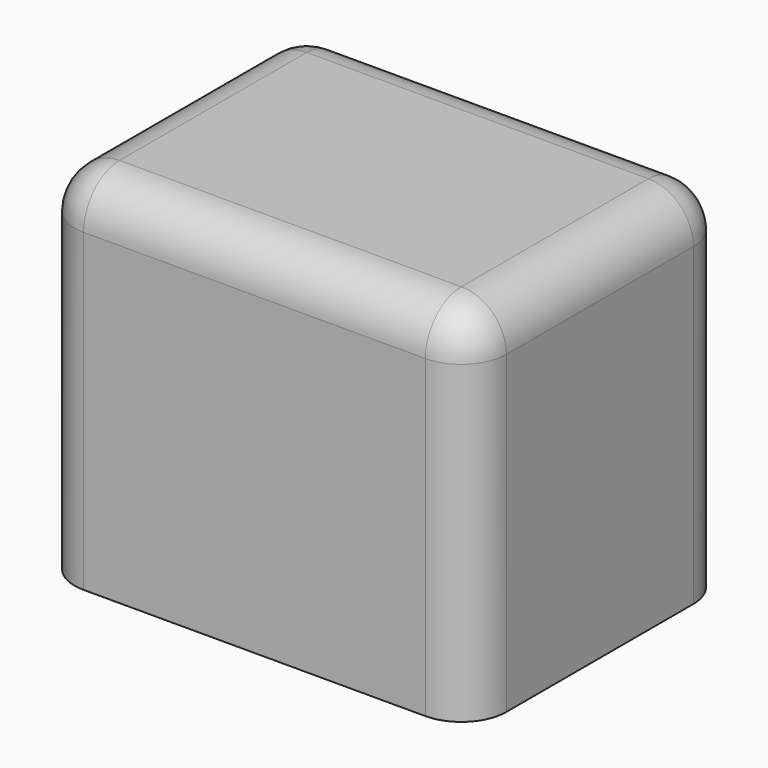
from build123d import *

# Parameters (mm, degrees)
F0_W     = 2.4
F0_H     = 2.4
F0_W_2   = 1.2
F0_H_2   = 1.2
F1_DEPTH = 7
F2_DEPTH = 1
F3_R     = 1


# Not quite as in the source:
# - a feature names something its author has since deleted; it is built from what else it names


with BuildPart() as f1:
    # F0 (on Top) → F1 (new body)
    with BuildSketch(Plane.XY):
        Polygon((-1.2, 6), (-1.2, 2.4), (-1.2, -1.2), (2.4, -1.2), (4.8, -1.2), (8.4, -1.2), (8.4, 2.4), (8.4, 6), (4.8, 6), (2.4, 6), align=None)
        Polygon((2.4, 0), (0, 0), (0, 2.4), (0, 4.8), (2.4, 4.8), (4.8, 4.8), (7.2, 4.8), (7.2, 2.4), (7.2, 0), (4.8, 0), align=None, mode=Mode.SUBTRACT)
        with Locations((1.2, 3.6)):
            Rectangle(F0_W, F0_H)
        with Locations((1.2, 3.6)):
            Rectangle(F0_W_2, F0_H_2, mode=Mode.SUBTRACT)
        with Locations((3.6, 3.6)):
            Rectangle(F0_W, F0_H)
        with Locations((3.6, 3.6)):
            Rectangle(F0_W_2, F0_H_2, mode=Mode.SUBTRACT)
        with Locations((6, 3.6)):
            Rectangle(F0_W, F0_H)
        with Locations((6, 3.6)):
            Rectangle(F0_W_2, F0_H_2, mode=Mode.SUBTRACT)
        with Locations((6, 1.2)):
            Rectangle(F0_W, F0_H)
        with Locations((6, 1.2)):
            Rectangle(F0_W_2, F0_H_2, mode=Mode.SUBTRACT)
        with Locations((3.6, 1.2)):
            Rectangle(F0_W, F0_H)
        with Locations((3.6, 1.2)):
            Rectangle(F0_W_2, F0_H_2, mode=Mode.SUBTRACT)
        with Locations((1.2, 1.2)):
            Rectangle(F0_W, F0_H)
        with Locations((1.2, 1.2)):
            Rectangle(F0_W_2, F0_H_2, mode=Mode.SUBTRACT)
    extrude(amount=-F1_DEPTH)

    # F0 (on Top) → F2 (join)
    with BuildSketch(Plane.XY):
        Polygon((-1.2, 6), (-1.2, 2.4), (-1.2, -1.2), (2.4, -1.2), (4.8, -1.2), (8.4, -1.2), (8.4, 2.4), (8.4, 6), (4.8, 6), (2.4, 6), align=None)
        Polygon((2.4, 0), (0, 0), (0, 2.4), (0, 4.8), (2.4, 4.8), (4.8, 4.8), (7.2, 4.8), (7.2, 2.4), (7.2, 0), (4.8, 0), align=None, mode=Mode.SUBTRACT)
        with Locations((3.6, 3.6)):
            Rectangle(F0_W, F0_H)
        with Locations((3.6, 3.6)):
            Rectangle(F0_W_2, F0_H_2, mode=Mode.SUBTRACT)
        with Locations((6, 3.6)):
            Rectangle(F0_W, F0_H)
        with Locations((6, 3.6)):
            Rectangle(F0_W_2, F0_H_2, mode=Mode.SUBTRACT)
        with Locations((1.2, 3.6)):
            Rectangle(F0_W, F0_H)
        with Locations((1.2, 3.6)):
            Rectangle(F0_W_2, F0_H_2, mode=Mode.SUBTRACT)
        with Locations((1.2, 1.2)):
            Rectangle(F0_W, F0_H)
        with Locations((1.2, 1.2)):
            Rectangle(F0_W_2, F0_H_2, mode=Mode.SUBTRACT)
        with Locations((3.6, 1.2)):
            Rectangle(F0_W, F0_H)
        with Locations((3.6, 1.2)):
            Rectangle(F0_W_2, F0_H_2, mode=Mode.SUBTRACT)
        with Locations((6, 1.2)):
            Rectangle(F0_W, F0_H)
        with Locations((6, 1.2)):
            Rectangle(F0_W_2, F0_H_2, mode=Mode.SUBTRACT)
        with Locations((6, 3.6)):
            Rectangle(F0_W_2, F0_H_2)
        with Locations((3.6, 3.6)):
            Rectangle(F0_W_2, F0_H_2)
        with Locations((1.2, 3.6)):
            Rectangle(F0_W_2, F0_H_2)
        with Locations((1.2, 1.2)):
            Rectangle(F0_W_2, F0_H_2)
        with Locations((3.6, 1.2)):
            Rectangle(F0_W_2, F0_H_2)
        with Locations((6, 1.2)):
            Rectangle(F0_W_2, F0_H_2)
    extrude(amount=F2_DEPTH)

    # F3
    f3_edges = [f1.edges().sort_by_distance(p)[0] for p in [
        (-1.2, -1.2, -3),
        (-1.2, 2.4, 1),
        (3.6, -1.2, 1),
        (8.4, -1.2, -3),
        (8.4, 2.4, 1),
        (3.6, 6, 1),
        (8.4, 6, -3),
        (-1.2, 6, -3),
    ]]
    fillet(f3_edges, radius=F3_R)


solid = f1.part
